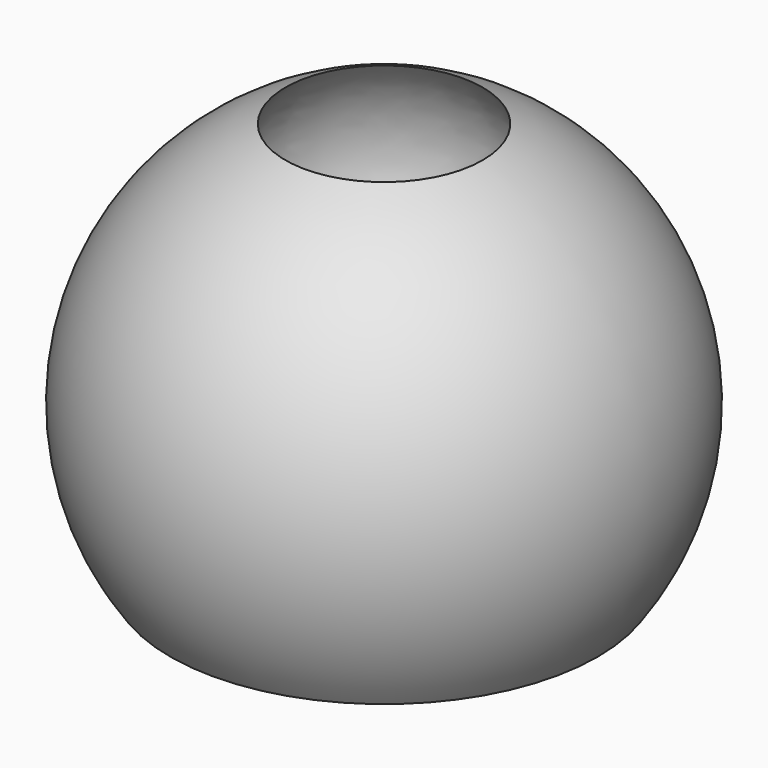
from build123d import *


with BuildPart() as f1:
    # F0 (on Front) → F1 (revolve)
    with BuildSketch(Plane.XZ):
        with BuildLine():
            Line((0, -35.9327479675), (49.6478166044, -35.9327479675))
            ThreePointArc((49.6478166044, -35.9327479675), (58.8880313325, 16.9784521045), (22.8972777039, 56.8487708207))
            ThreePointArc((22.8972777039, 56.8487708207), (30.4760832971, 20.7606017759), (0, 0))
            Line((0, 0), (0, -35.9327479675))
        make_face()
    revolve(axis=Axis((0, 0, 15.8958256506), (0, 0, 1)))


solid = f1.part
